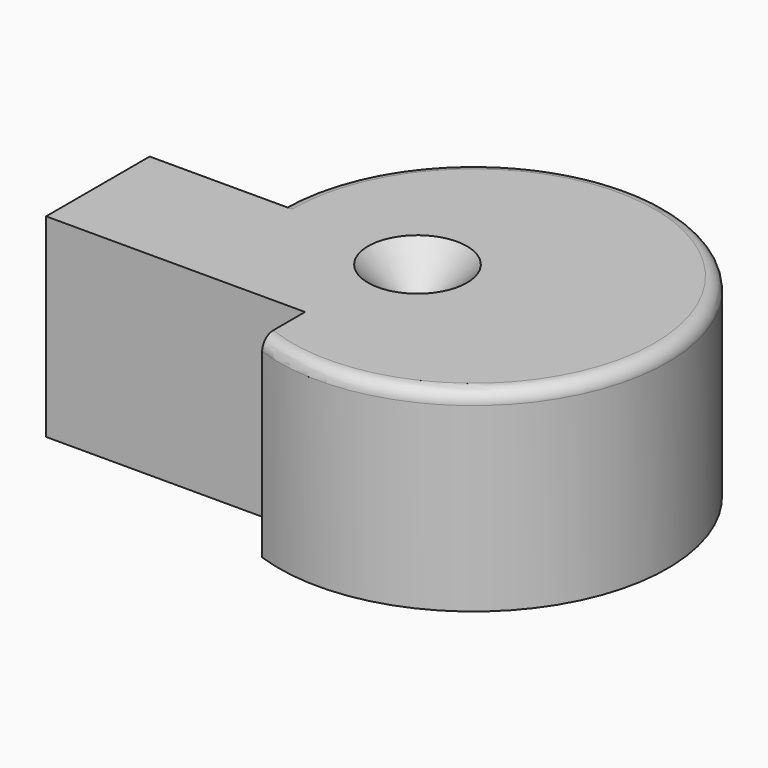
from build123d import *

# Parameters (mm, degrees)
F1_DEPTH = 76.2
F2_R     = 5.08
F3_R     = 19.4175013285


# Not quite as in the source:
# - an extrude whose draft closes it to a point is written as a loft to that point


with BuildPart() as f1:
    # F0 (on Top) → F1 (new body)
    with BuildSketch(Plane.XY):
        with BuildLine():
            Line((0, 50.8), (0, 0))
            Line((0, 0), (101.6, 0))
            Line((101.6, 0), (101.6, -21.0420489686))
            ThreePointArc((101.6, -21.0420489686), (189.2170394667, 94.7940905122), (50.8, 50.8))
            Line((50.8, 50.8), (0, 50.8))
        make_face()
    extrude(amount=F1_DEPTH)

    # F2
    f2_edges = [f1.edges().sort_by_distance(p)[0] for p in [
        (189.217039, 94.794091, 76.2),
    ]]
    fillet(f2_edges, radius=F2_R)

    # F3 (on face) → F4 section 0
    with BuildSketch(Plane.XY.offset(76.2), mode=Mode.PRIVATE) as f4_s0:
        with Locations((108.8073253632, 46.1364276707)):
            Circle(F3_R)
    loft([f4_s0.sketch, Vertex(108.8073253632, 46.1364276707, 56.7824986715)], ruled=True, mode=Mode.SUBTRACT)


solid = f1.part
